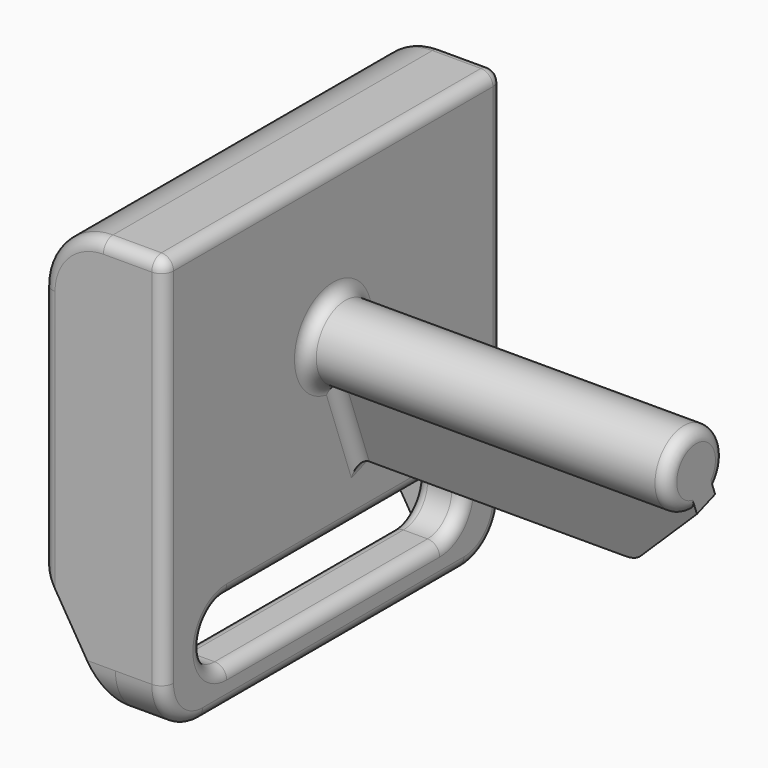
from build123d import *

# Parameters (mm, degrees)
F0_W      = 35
F0_H      = 25
F1_DEPTH  = 6
F3_DEPTH  = 4
F4_R      = 1
F6_DEPTH  = 6
F8_DEPTH  = 35.001
F10_DEPTH = 30
F11_SIZE  = 7
F12_R     = 2
F13_R     = 5
F14_R     = 1
F15_R     = 1


with BuildPart() as f1:
    # F0 (on Right) → F1 (new body)
    with BuildSketch(Plane.YZ):
        Rectangle(F0_W, F0_H)
    extrude(amount=F1_DEPTH)

    # F2 (on face) → F3 (join)
    with BuildSketch(Plane.YZ.offset(6)):
        with BuildLine():
            Line((17.5, 12.5), (-17.5, 12.5))
            Line((-17.5, 12.5), (-17.5, -18.5))
            ThreePointArc((-17.5, -18.5), (-16.3284271247, -21.3284271247), (-13.5, -22.5))
            Line((-13.5, -22.5), (13.5, -22.5))
            ThreePointArc((13.5, -22.5), (16.3284271247, -21.3284271247), (17.5, -18.5))
            Line((17.5, -18.5), (17.5, 12.5))
        make_face()
        with BuildLine():
            ThreePointArc((-11, -19.5), (-13.5, -17), (-11, -14.5))
            Line((-11, -14.5), (11, -14.5))
            ThreePointArc((11, -14.5), (13.5, -17), (11, -19.5))
            Line((11, -19.5), (-11, -19.5))
        make_face(mode=Mode.SUBTRACT)
    extrude(amount=F3_DEPTH)

    # F4
    f4_edges = [f1.edges().sort_by_distance(p)[0] for p in [
        (10, -16.328427, -21.328427),
        (10, 0, -19.5),
        (6, 0, -19.5),
    ]]
    fillet(f4_edges, radius=F4_R)

    # F5 (on face) → F6 (join, through all)
    with BuildSketch(Plane(origin=(6, 0, 0), x_dir=(0, -1, 0), z_dir=(-1, 0, 0))):
        with BuildLine():
            Line((17.5, -12.5), (14.5, -12.5))
            Line((14.5, -12.5), (14.5, -22.3729833462))
            ThreePointArc((14.5, -22.3729833462), (16.6622776602, -20.9494897428), (17.5, -18.5))
            Line((17.5, -18.5), (17.5, -12.5))
        make_face()
        with BuildLine():
            Line((-14.5, -12.5), (-17.5, -12.5))
            Line((-17.5, -12.5), (-17.5, -18.5))
            ThreePointArc((-17.5, -18.5), (-16.6622776602, -20.9494897428), (-14.5, -22.3729833462))
            Line((-14.5, -22.3729833462), (-14.5, -12.5))
        make_face()
    extrude(amount=F6_DEPTH)

    # F7 (on face) → F8 (cut, through all)
    with BuildSketch(Plane.XZ.offset(17.5)):
        Polygon((6, -22.3729833462), (0, -12.5), (0, -22.3729833462), align=None)
    extrude(amount=-F8_DEPTH, mode=Mode.SUBTRACT)

    # F9 (on face) → F10 (join)
    with BuildSketch(Plane.YZ.offset(10)):
        with BuildLine():
            Line((4.359894054, -9.0739122182), (1.9070716714, -2.3348381079))
            ThreePointArc((1.9070716714, -2.3348381079), (-1.02606043, 2.8000717087), (0.0276864298, -3.0188783946))
            Line((0.0276864298, -3.0188783946), (2.4805088125, -9.7579525049))
            Line((2.4805088125, -9.7579525049), (4.359894054, -9.0739122182))
        make_face()
    extrude(amount=F10_DEPTH)

    # F11
    f11_edges = [f1.edges().sort_by_distance(p)[0] for p in [
        (40, 3.420201, -9.415932),
    ]]
    chamfer(f11_edges, length=F11_SIZE)

    # F12
    f12_edges = [f1.edges().sort_by_distance(p)[0] for p in [
        (33, 3.420201, -9.415932),
    ]]
    fillet(f12_edges, radius=F12_R)

    # F13
    f13_edges = [f1.edges().sort_by_distance(p)[0] for p in [
        (0, 0, 12.5),
    ]]
    fillet(f13_edges, radius=F13_R)

    # F14
    f14_edges = [f1.edges().sort_by_distance(p)[0] for p in [
        (0, 17.5, -2.5),
    ]]
    fillet(f14_edges, radius=F14_R)

    # F15
    f15_edges = [f1.edges().sort_by_distance(p)[0] for p in [
        (10, 3.133483, -5.704375),
        (10, -1.02606, 2.800072),
        (10, 3.420201, -9.415932),
        (10, 1.254098, -6.388415),
        (40, -1.02606, 2.800072),
    ]]
    fillet(f15_edges, radius=F15_R)


solid = f1.part
